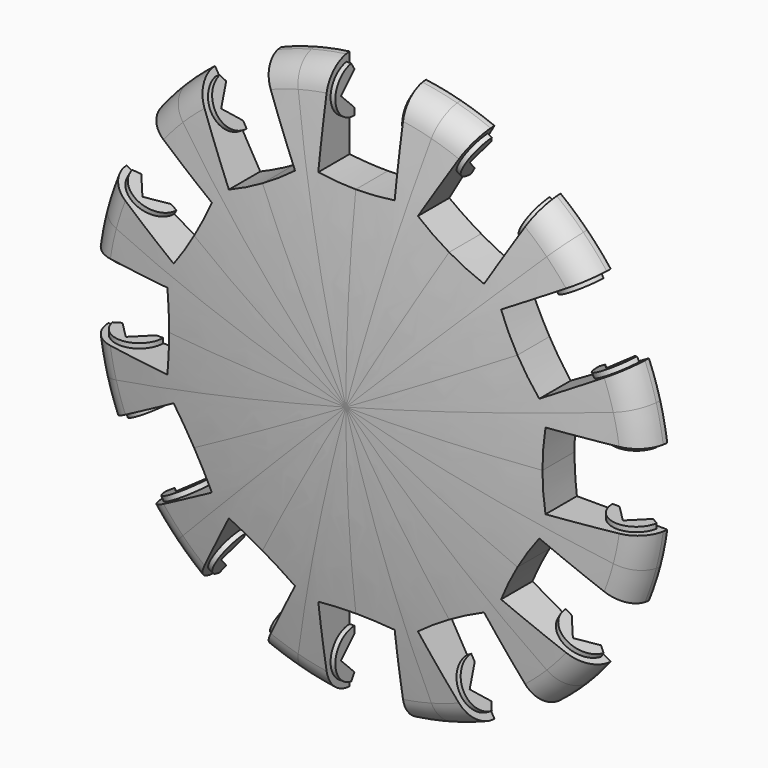
from build123d import *
from build123d import SkipClean  # not in build123d's __all__

# Parameters (mm, degrees)
F2_DEPTH  = 2.2
F4_DEPTH  = 1.4582128393
F6_ANGLE  = 30
F8_DEPTH  = 0.2
F10_COUNT = 12


with BuildPart() as f2:
    # F1 (on Front) → F2 (new body)
    with BuildSketch(Plane.XZ):
        with BuildLine():
            ThreePointArc((1.6, 7.9181845537), (0.8015249223, 7.8440801349), (0, 7.819347292))
            Line((0, 7.819347292), (0, 0))
            Line((0, 0), (3.0572128393, 11.409673646))
            Line((3.0572128393, 11.409673646), (1.6, 11.8001326495))
            Line((1.6, 11.8001326495), (1.6, 11.409673646))
            Line((1.6, 11.409673646), (1.6, 7.9181845537))
        make_face()
    extrude(amount=F2_DEPTH)

    # F3 (on face) → F4 (cut, through all)
    with BuildSketch(Plane(origin=(1.6, 0, 0), x_dir=(0, -1, 0), z_dir=(-1, 0, 0))):
        Polygon((0.7071067812, 10.409673646), (0, 11.1167804272), (0, 9.7025668648), align=None)
    extrude(amount=-F4_DEPTH, mode=Mode.SUBTRACT)

    # F5 (on face) → F6 (revolve, cut)
    with BuildSketch(Plane(origin=(0, 0, 0), x_dir=(0, 1, 0), z_dir=(0.9659258263, 0, -0.2588190451))):
        with BuildLine():
            ThreePointArc((-2.2, 0), (-1.9512521734, 5.4112645022), (-1.2071067812, 10.7768871715))
            ThreePointArc((-1.2071067812, 10.7768871715), (-0.8558422622, 11.4439242872), (-0.188619393, 11.7948358413))
            ThreePointArc((-0.188619393, 11.7948358413), (-0.0947068082, 11.8078223733), (0, 11.8121633519))
            Line((0, 11.8121633519), (0, 12.9670836031))
            Line((0, 12.9670836031), (-2.2, 12.9670836031))
            Line((-2.2, 12.9670836031), (-2.2, 11.8121633519))
            Line((-2.2, 11.8121633519), (-2.2, 0))
        make_face()
    revolve(axis=Axis((0, -1.1, 0), (0, -1, 0)), revolution_arc=F6_ANGLE, mode=Mode.SUBTRACT)

    # F7 (on face) → F8 (join)
    with BuildSketch(Plane(origin=(1.6, 0, 0), x_dir=(0, -1, 0), z_dir=(-1, 0, 0))):
        with BuildLine():
            Line((0, 9.7025668648), (0, 9.409673646))
            ThreePointArc((0, 9.409673646), (0.9964799699, 10.3258424487), (0.167072218, 11.3956183067))
            Line((0.167072218, 11.3956183067), (0, 11.1167804272))
            Line((0, 11.1167804272), (0.7071067812, 10.409673646))
            Line((0.7071067812, 10.409673646), (0, 9.7025668648))
        make_face()
    extrude(amount=F8_DEPTH)

    # F9: F2 across face


with BuildPart() as f2_1:
    add(f2.part, clean=False)
    with SkipClean():  # cleaning this boolean's faces spoils the solid; the shape is the same uncleaned
        add(f2.part.mirror(Plane(origin=(1.3070018383, -0.9555401299, 4.8777972662), x_dir=(0, 1, 0), z_dir=(0.9659258263, 0, -0.2588190451))), clean=False)

    # F10: F2 ×12 about axis
    f10_axis = Axis((0, -1.1, 0), (0, 1, 0))


with BuildPart() as f2_2:
    add(f2_1.part, clean=False)
    with SkipClean():  # cleaning this boolean's faces spoils the solid; the shape is the same uncleaned
        for i in range(1, F10_COUNT):
            add(f2_1.part.rotate(f10_axis, i * 360 / F10_COUNT), clean=False)


solid = f2_2.part
